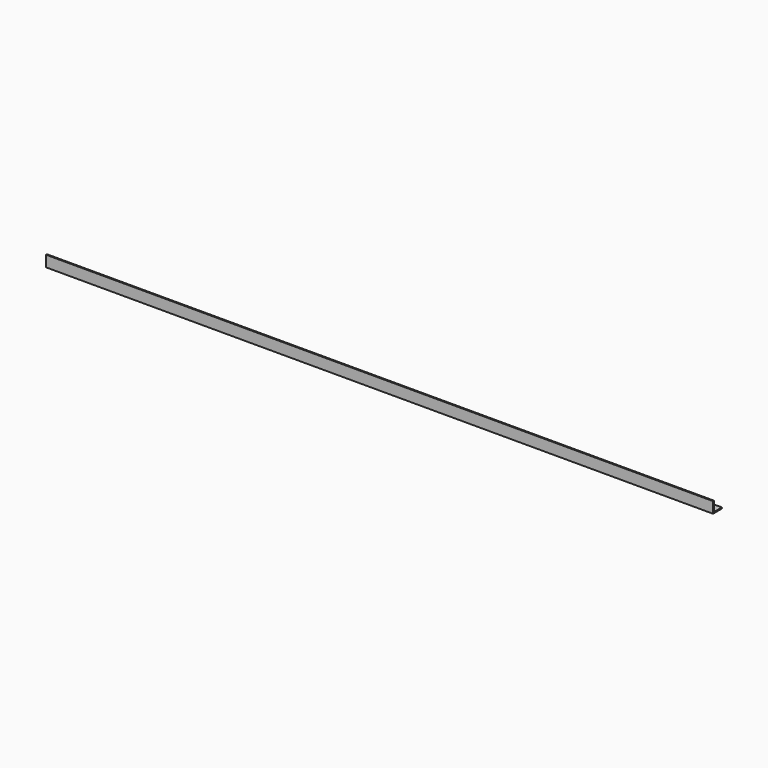
from build123d import *

# Parameters (mm, degrees)
F1_DEPTH = 6000
F3_D     = 22


with BuildPart() as f1:
    # F0 (on Right) → F1 (new body)
    with BuildSketch(Plane.YZ):
        Polygon((0, 100), (0, 0), (100, 0), (100, 10), (10, 10), (10, 100), align=None)
    extrude(amount=F1_DEPTH)

    # F3 (through all)
    with Locations(Plane(origin=(0, 0, 0), x_dir=(1, 0, 0), z_dir=(0, 0, -1))):
        with Locations((75, -55.9013597667)):
            Hole(F3_D / 2)


solid = f1.part
